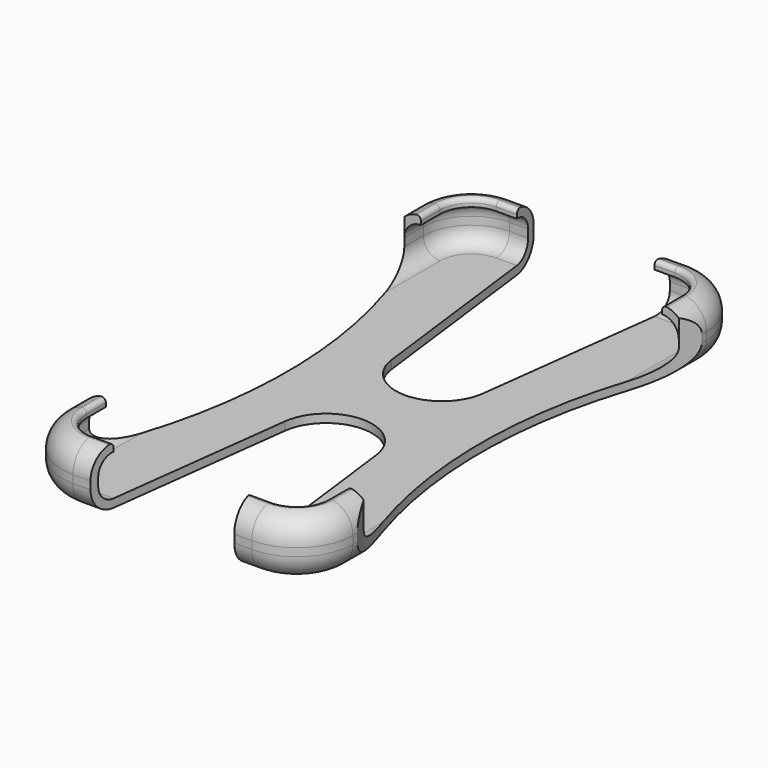
from build123d import *

# Parameters (mm, degrees)
F1_DEPTH = 17.653
F2_R     = 7.62
F3_T     = -2.54
F5_DEPTH = 17.654
F7_DEPTH = 17.654
F8_W     = 34.620501101
F8_H     = 14.1270561144
F9_DEPTH = 53.09035
F10_R    = 1.27


# Not quite as in the source:
# - a shell that OpenCascade refuses in one call is made with other operations: the cavity is built on its own and cut out


with BuildPart() as f1:
    # F0 (on Top) → F1 (new body)
    with BuildSketch(Plane.XY):
        with BuildLine():
            Line((27.305, 84.582), (-27.305, 84.582))
            ThreePointArc((-27.305, 84.582), (-39.4283457634, 79.5603457634), (-44.45, 67.437))
            Line((-44.45, 67.437), (-44.45, -67.437))
            ThreePointArc((-44.45, -67.437), (-39.4283457634, -79.5603457634), (-27.305, -84.582))
            Line((-27.305, -84.582), (27.305, -84.582))
            ThreePointArc((27.305, -84.582), (39.4283457634, -79.5603457634), (44.45, -67.437))
            Line((44.45, -67.437), (44.45, 67.437))
            ThreePointArc((44.45, 67.437), (39.4283457634, 79.5603457634), (27.305, 84.582))
        make_face()
    extrude(amount=F1_DEPTH)

    # F2
    f2_edges = [f1.edges().sort_by_distance(p)[0] for p in [
        (0, 84.582, 17.653),
        (-39.428346, 79.560346, 17.653),
        (-44.45, 0, 17.653),
        (-39.428346, -79.560346, 17.653),
        (0, -84.582, 17.653),
        (39.428346, -79.560346, 17.653),
        (44.45, 0, 17.653),
        (39.428346, 79.560346, 17.653),
        (0, 84.582, 0),
        (-39.428346, 79.560346, 0),
        (-44.45, 0, 0),
        (-39.428346, -79.560346, 0),
        (0, -84.582, 0),
        (39.428346, -79.560346, 0),
        (44.45, 0, 0),
        (39.428346, 79.560346, 0),
    ]]
    fillet(f2_edges, radius=F2_R)

    # F3: a shell. OpenCascade refuses it in one call, so the cavity is built on its own and cut out:
    # the body offset inwards by the wall thickness, plus a prism from it out through each open face.
    f3_core = offset(f1.part, amount=F3_T, mode=Mode.PRIVATE)
    f3_exits = [f3_core.faces().sort_by_distance(p)[0] for p in [
        (0, 0, 15.113),
    ]]
    add(f3_core, mode=Mode.SUBTRACT)
    extrude(f3_exits, amount=-F3_T, mode=Mode.SUBTRACT)

    # F4 (on Top) → F5 (cut, through all)
    with BuildSketch(Plane.XY):
        with BuildLine():
            Line((-22.4742740393, 88.7566655874), (-13.9317430833, 20.3375323037))
            ThreePointArc((-13.9317430833, 20.3375323037), (0, 8.0370782698), (13.9317430833, 20.3375323037))
            Line((13.9317430833, 20.3375323037), (22.4742740393, 88.7566655874))
            Line((22.4742740393, 88.7566655874), (-22.4742740393, 88.7566655874))
        make_face()
        with BuildLine():
            Line((-13.9317430833, -20.3375323037), (-22.4742740393, -88.7566655874))
            Line((-22.4742740393, -88.7566655874), (22.4742740393, -88.7566655874))
            Line((22.4742740393, -88.7566655874), (13.9317430833, -20.3375323037))
            ThreePointArc((13.9317430833, -20.3375323037), (0, -8.0370782698), (-13.9317430833, -20.3375323037))
        make_face()
    extrude(amount=F5_DEPTH, mode=Mode.SUBTRACT)

    # F6 (on Top) → F7 (cut, through all)
    with BuildSketch(Plane.XY):
        with BuildLine():
            Line((53.8405366242, -82.55), (53.8405366242, 82.55))
            ThreePointArc((53.8405366242, 82.55), (29.5469669858, 0), (53.8405366242, -82.55))
        make_face()
        with BuildLine():
            ThreePointArc((-53.8405366242, -82.55), (-29.5469669858, 0), (-53.8405366242, 82.55))
            Line((-53.8405366242, 82.55), (-53.8405366242, -82.55))
        make_face()
    extrude(amount=F7_DEPTH, mode=Mode.SUBTRACT)

    # F8 (on Right) → F9 (cut, symmetric)
    with BuildSketch(Plane.YZ):
        with Locations((-42.8180113353, 14.6059473045)):
            Rectangle(F8_W, F8_H)
        with Locations((42.8180113353, 14.6059473045)):
            Rectangle(F8_W, F8_H)
    extrude(amount=F9_DEPTH, both=True, mode=Mode.SUBTRACT)

    # F10
    f10_edges = [f1.edges().sort_by_distance(p)[0] for p in [
        (-34.040192, 74.172192, 17.653),
        (-34.040192, -74.172192, 17.653),
        (34.040192, -74.172192, 17.653),
        (34.040192, 74.172192, 17.653),
    ]]
    fillet(f10_edges, radius=F10_R)


solid = f1.part
